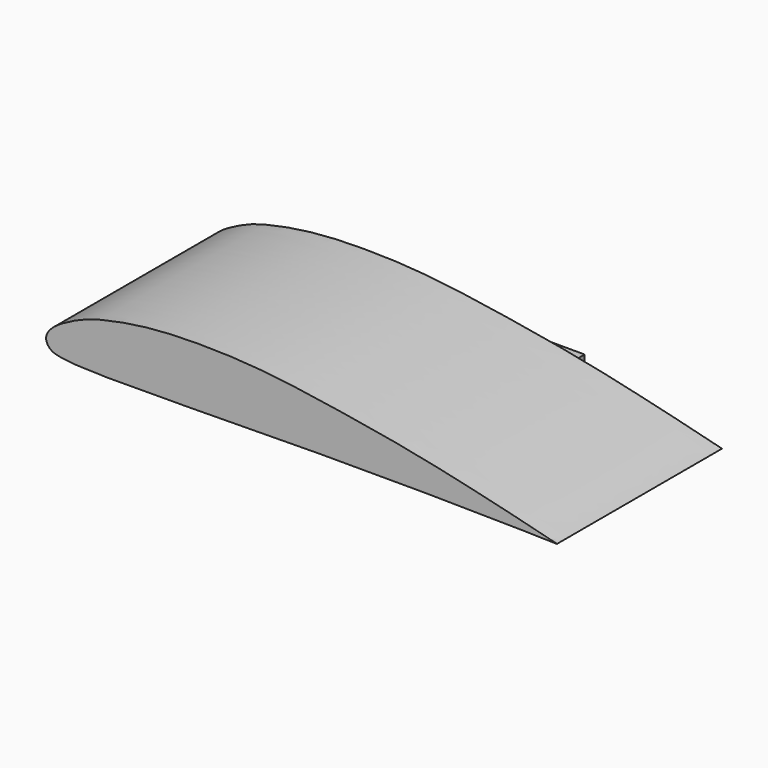
from build123d import *

# Parameters (mm, degrees)
F0_W     = 19.05
F0_H     = 6.35
F1_DEPTH = 76.2
F2_DEPTH = 6.35


# Not quite as in the source:
# - the dataset's text gives a spline's control points without its knots; the knots are read off the source's solid


with BuildPart() as f1:
    # F0 (on Front) → F1 (new body)
    with BuildSketch(Plane.XZ):
        with BuildLine():
            add(Edge.make_bspline(
                [(113.1256508208, -7.7402851731), (113.097200705, -7.8031856437), (110.3364793373, -7.6968863686), (99.3152862089, -7.4328909753), (55.9796904977, -6.7675201656), (16.8725827, -7.0164671979), (15.6765189296, -7.0293432408), (-47.4697706514, -7.9806912282), (-59.2372081566, -7.5517426686), (-66.7167856923, -7.3252423551), (-71.4929241921, -6.5336386662), (-72.7223444909, -6.1638428264), (-73.4842272273, -5.8153616349), (-74.1766086139, -5.3340215063), (-74.7800065829, -4.7393990674), (-75.2101915382, -4.1532632538), (-75.5045783983, -3.6131817045), (-75.687252981, -3.0871754263), (-75.7613287218, -2.7553238198), (-75.8086858659, -2.2774327515), (-75.7716160209, -1.7899042913), (-75.6387924297, -1.2158513369), (-75.3863023669, -0.5591157083), (-74.7985947775, 0.4212869121), (-73.9676114059, 1.4201144876), (-72.4438088281, 2.8224936522), (-69.9908402735, 4.4607384308), (-65.3335290261, 6.9575761188), (-60.68863408, 8.9396673965), (-55.5979076782, 10.3985471041), (-48.0040197216, 12.0564073917), (-39.7134136622, 13.3073162495), (-30.4791055277, 14.086241923), (-19.9483485157, 14.3421894431), (-7.3587359983, 14.1261353089), (4.8627801197, 13.2128038161), (17.447836634, 11.7218204499), (37.3969921311, 8.6625017009), (57.7235038813, 5.1464122385), (75.7922924691, 1.3014360791), (97.7888660124, -3.8123268572), (110.2840958287, -7.0876782322), (113.154565826, -7.6763568769), (113.1256508208, -7.7402851731)],
                knots=[0, 0, 0, 0, 0.0130491957, 0.0440066043, 0.1109645612, 0.1693650629, 0.1845200279, 0.2601585935, 0.297227308, 0.3222519534, 0.3432259075, 0.3538117117, 0.3623972714, 0.3712966115, 0.3802460949, 0.3885022479, 0.3961575709, 0.4032942665, 0.4089630871, 0.4155815182, 0.42240654, 0.4297507891, 0.4378777956, 0.4481278983, 0.459205589, 0.4728705156, 0.4895752088, 0.5119006412, 0.5337815859, 0.555985693, 0.5829463887, 0.6112137679, 0.6406139011, 0.6721764069, 0.7067075957, 0.7404524036, 0.7749091572, 0.8185379831, 0.8627452602, 0.9048194685, 0.9516457096, 0.9867375738, 1, 1, 1, 1], degree=3))
        make_face()
        with Locations((-55.4735022347, -0.4073630356)):
            Rectangle(F0_W, F0_H, mode=Mode.SUBTRACT)
        with Locations((47.7571423614, -0.9834326582)):
            Rectangle(F0_W, F0_H, mode=Mode.SUBTRACT)
        with Locations((-4.6735022347, 4.9266369644)):
            Rectangle(F0_W, F0_H, mode=Mode.SUBTRACT)
        with Locations((-55.4735022347, -0.4073630356)):
            Rectangle(F0_W, F0_H)
        with Locations((-4.6735022347, 4.9266369644)):
            Rectangle(F0_W, F0_H)
        with Locations((47.7571423614, -0.9834326582)):
            Rectangle(F0_W, F0_H)
    extrude(amount=F1_DEPTH)

    # F0 (on Front) → F2 (join)
    with BuildSketch(Plane.XZ):
        with Locations((-55.4735022347, -0.4073630356)):
            Rectangle(F0_W, F0_H)
        with Locations((-4.6735022347, 4.9266369644)):
            Rectangle(F0_W, F0_H)
        with Locations((47.7571423614, -0.9834326582)):
            Rectangle(F0_W, F0_H)
    extrude(amount=-F2_DEPTH)


solid = f1.part
